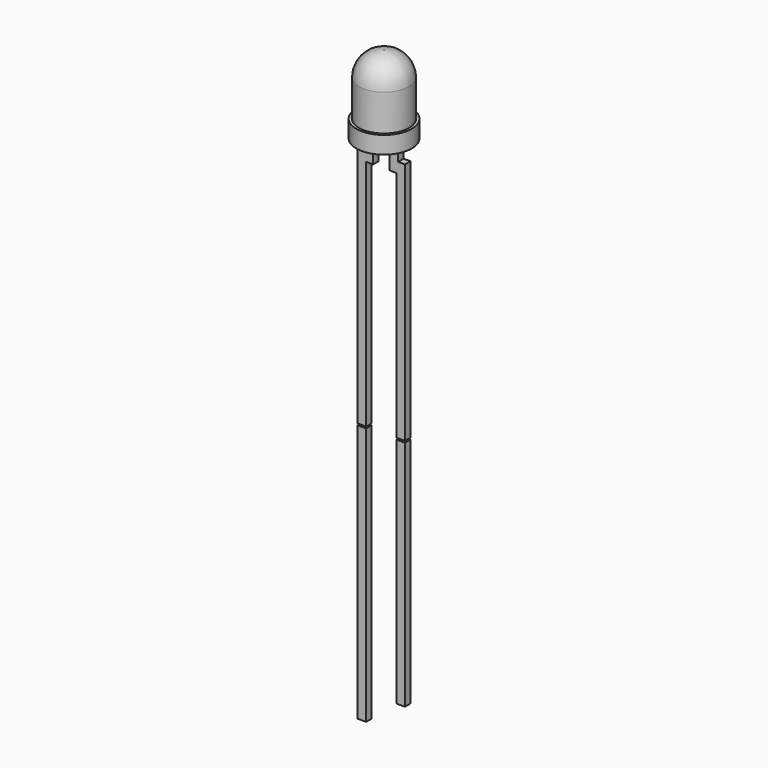
from build123d import *

# Parameters (mm, degrees)
F2_DEPTH = 0.2
F0_W     = 0.5
F0_H     = 0.1
F3_DEPTH = 0.2
F0_H_2   = 14.9325303316
F4_DEPTH = 0.2
F0_H_3   = 13.4325303316


# Not quite as in the source:
# - the program builds the solid bodies; features that only make, move or delete a surface that nothing else refers to are left out


with BuildPart() as f1:
    # F0 (on Front) → F1 (revolve)
    with BuildSketch(Plane.XZ):
        with BuildLine():
            Line((0, 1), (1.45, 1))
            Line((1.45, 1), (1.45, 3.1))
            ThreePointArc((1.45, 3.1), (1.0399494937, 4.0899494937), (0.05, 4.5))
            Line((0.05, 4.5), (0, 4.5))
            Line((0, 4.5), (0, 1))
        make_face()
        Polygon((1.6, 0), (1.6, 1), (1.45, 1), (0, 1), (0, 0), (0.3817705219, 0), (0.47, 0), (0.97, 0), (1.0582294781, 0), align=None)
    revolve(axis=Axis((0, 0, 2.75), (0, 0, 1)))

    # F0 (on Front) → F2 (join, symmetric)
    with BuildSketch(Plane.XZ):
        Polygon((0.97, -0.65), (0.97, 0), (0.47, 0), (0.47, -0.65), (0.47, -1.4), (0.87, -1.4), (0.87, -14.8674696684), (1.37, -14.8674696684), (1.37, -0.8), (0.97, -0.8), align=None)
        Polygon((-0.47, -0.65), (-0.47, 0), (-0.97, 0), (-0.97, -0.65), (-0.97, -0.8), (-1.37, -0.8), (-1.37, -14.8674696684), (-0.87, -14.8674696684), (-0.87, -1.4), (-0.47, -1.4), align=None)
    extrude(amount=F2_DEPTH, both=True)

    # F0 (on Front) → F3 (cut, symmetric)
    with BuildSketch(Plane.XZ):
        with Locations((1.12, -14.9174696684)):
            Rectangle(F0_W, F0_H)
        with Locations((-1.12, -14.9174696684)):
            Rectangle(F0_W, F0_H)
    extrude(amount=F3_DEPTH, both=True, mode=Mode.SUBTRACT)


with BuildPart() as f4:
    # F0 (on Front) → F4 (new body, symmetric)
    with BuildSketch(Plane.XZ):
        with Locations((-1.12, -22.4337348342)):
            Rectangle(F0_W, F0_H_2)
    extrude(amount=F4_DEPTH, both=True)


with BuildPart() as f4b:
    # F0 (on Front) → F4, piece 2 (new body, symmetric)
    with BuildSketch(Plane.XZ):
        with Locations((1.12, -21.6837348342)):
            Rectangle(F0_W, F0_H_3)
    extrude(amount=F4_DEPTH, both=True)


solid = Compound([f1.part, f4.part, f4b.part])
